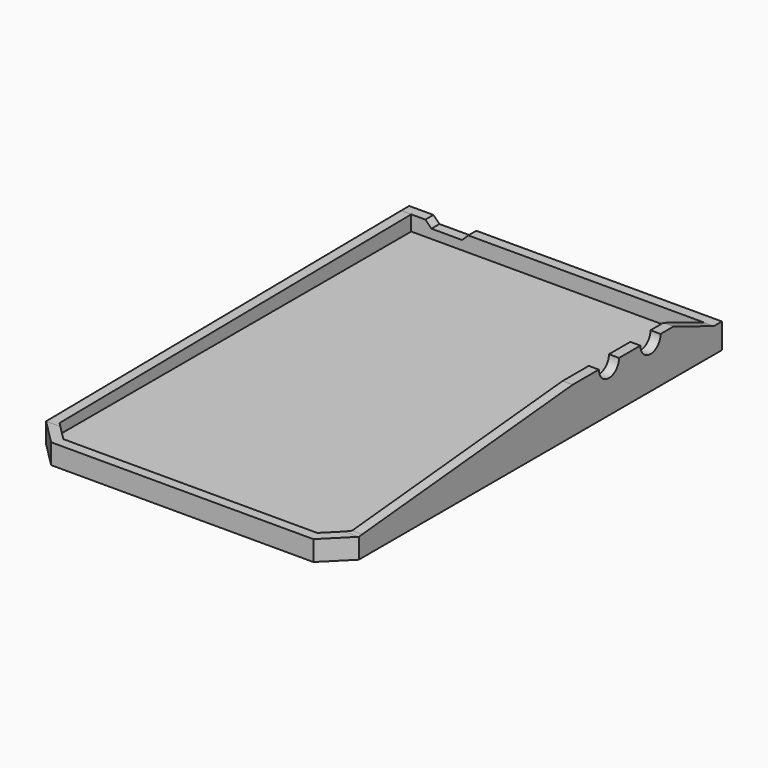
from build123d import *

# Parameters (mm, degrees)
F0_W      = 62
F0_H      = 95
F1_DEPTH  = 9
F2_SIZE   = 5
F3_T      = -2
F5_DEPTH  = 2
F7_DEPTH  = 2
F8_DEPTH  = 25
F10_DEPTH = 90
F12_DEPTH = 3


with BuildPart() as f1:
    # F0 (on Top) → F1 (new body)
    with BuildSketch(Plane.XY):
        Rectangle(F0_W, F0_H)
    extrude(amount=F1_DEPTH)

    # F2
    f2_edges = [f1.edges().sort_by_distance(p)[0] for p in [
        (-31, -47.5, 4.5),
        (31, -47.5, 4.5),
    ]]
    chamfer(f2_edges, length=F2_SIZE)

    # F3
    f3_openings = [f1.faces().sort_by_distance(p)[0] for p in [
        (0, 0.195368, 9),
    ]]
    offset(amount=F3_T, openings=f3_openings)

    # F4 (on face) → F5 (cut)
    with BuildSketch(Plane.YZ.offset(31)):
        with BuildLine():
            ThreePointArc((27.3, 9), (29.8, 6.5), (32.3, 9))
            Line((32.3, 9), (35.5, 9))
            Line((35.5, 9), (45.5, 5))
            Line((45.5, 5), (47.5, 5))
            Line((47.5, 5), (47.5, 10))
            Line((47.5, 10), (-47.5, 10))
            Line((-47.5, 10), (-47.5, 4))
            Line((-47.5, 4), (-42.5, 4))
            Line((-42.5, 4), (10.5, 9))
            Line((10.5, 9), (17, 9))
            ThreePointArc((17, 9), (19.5, 6.5), (22, 9))
            Line((22, 9), (27.3, 9))
        make_face()
    extrude(amount=-F5_DEPTH, mode=Mode.SUBTRACT)

    # F6 (on face) → F7 (cut)
    with BuildSketch(Plane(origin=(0, 47.5, 0), x_dir=(-1, 0, 0), z_dir=(0, 1, 0))):
        Polygon((-29, 9), (-29, 5), (-25.9392373264, 5), (17.7, 5), (18.9, 3.8), (25, 3.8), (26.2, 5), (31, 5), (31, 9), align=None)
    extrude(amount=-F7_DEPTH, mode=Mode.SUBTRACT)

    # F8 (add): a face of the model
    f8_faces = [f1.faces().sort_by_distance(p)[0] for p in [
        (29, -43.0883975313, 6.5056760177),
    ]]
    extrude(f8_faces, amount=F8_DEPTH)

    # F9 (on face) → F10 (cut)
    with BuildSketch(Plane.YZ.offset(54)):
        Polygon((-42.5, 4), (-41.6715728753, 4.0781535023), (-41.6715728753, 9.3699973077), (-47.5018471479, 9.3699973077), (-47.5018471479, 4), align=None)
    extrude(amount=-F10_DEPTH, mode=Mode.SUBTRACT)

    # F11 (on face) → F12 (cut)
    with BuildSketch(Plane(origin=(-31, 0, 0), x_dir=(0, -1, 0), z_dir=(-1, 0, 0))):
        Polygon((-45.5, 9), (-45.5, 5), (42.5, 4), (42.5568181818, 9), align=None)
    extrude(amount=-F12_DEPTH, mode=Mode.SUBTRACT)


solid = f1.part
